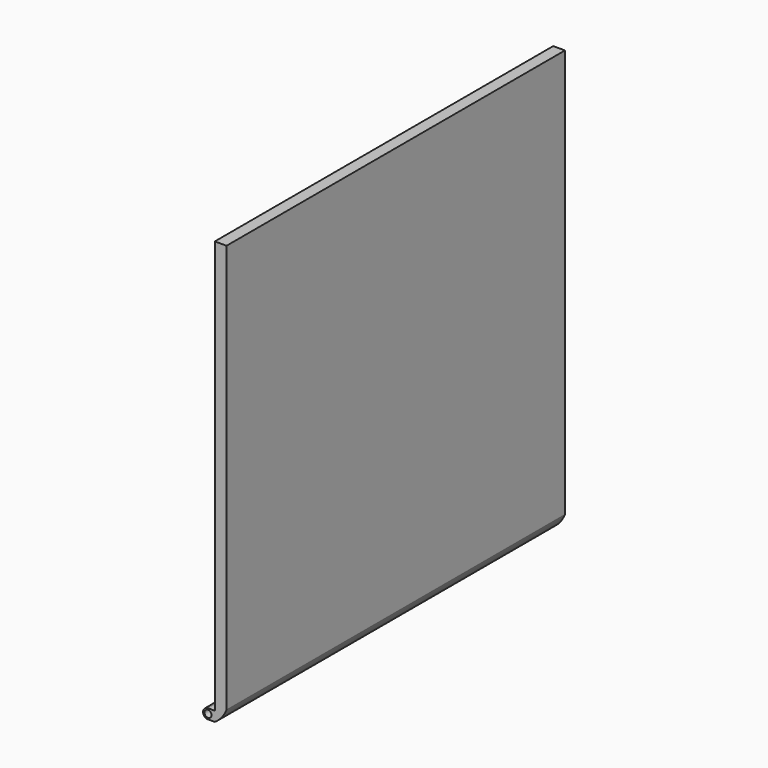
from build123d import *

# Parameters (mm, degrees)
F0_W     = 914.4
F0_H     = 914.4
F1_DEPTH = 25.4
F2_R     = 7.62
F3_DEPTH = 457.2
F5_DEPTH = 914.4


with BuildPart() as f1:
    # F0 (on Right) → F1 (new body)
    with BuildSketch(Plane.YZ):
        Rectangle(F0_W, F0_H)
    extrude(amount=F1_DEPTH)

    # F2 (on Front) → F3 (join, through all)
    with BuildSketch(Plane.XZ):
        with BuildLine():
            Line((0, -435.864), (-14.732, -435.864))
            ThreePointArc((-14.732, -435.864), (-25.4, -446.532), (-14.732, -457.2))
            Line((-14.732, -457.2), (0, -457.2))
            Line((0, -457.2), (0, -435.864))
        make_face()
        with Locations((-14.732, -446.532)):
            Circle(F2_R, mode=Mode.SUBTRACT)
    extrude(amount=F3_DEPTH)

    # F4 (on face) → F5 (cut, through all)
    with BuildSketch(Plane.XZ.offset(457.2)):
        with BuildLine():
            ThreePointArc((25.4, -425.6636202335), (15.2344848329, -443.4731324002), (0, -457.2))
            Line((0, -457.2), (25.4, -457.2))
            Line((25.4, -457.2), (25.4, -425.6636202335))
        make_face()
    extrude(amount=-F5_DEPTH, mode=Mode.SUBTRACT)


solid = f1.part
